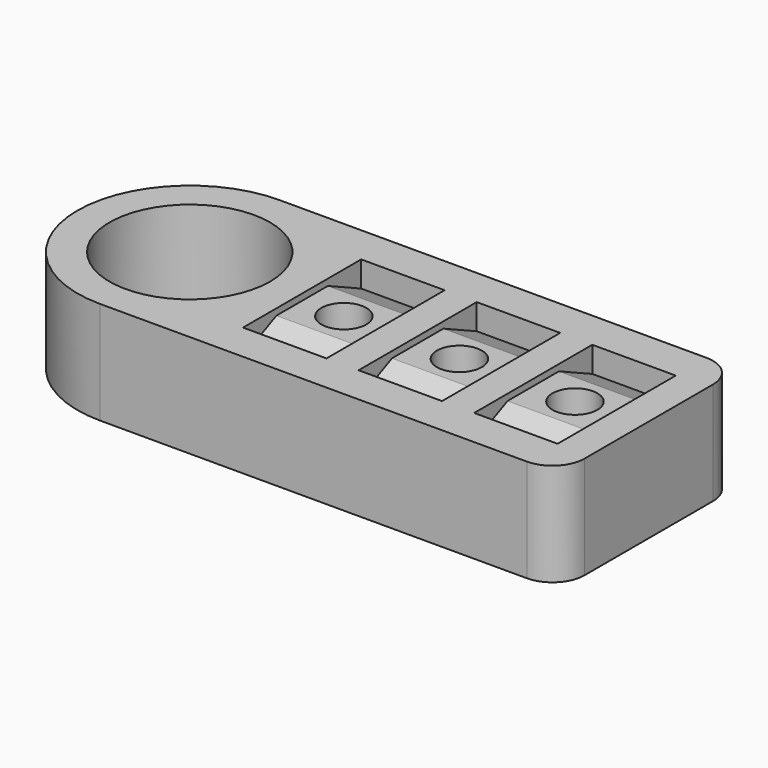
from build123d import *

# Parameters (mm, degrees)
F0_R         = 12.5
F1_DEPTH     = 16
F3_START     = -5
F3_DEPTH     = 13
F4_START     = -23
F4_DEPTH     = 13
F5_START     = -41
F5_DEPTH     = 13
F6_R         = 3.5
F7_DEPTH     = 14
F8_TEXT_SIZE = 5.5555555556
F9_DEPTH     = 1


# Not quite as in the source:
# - Text() gives the source's letters only with a copy of the font that has no kerning and outlines rounded to 1/6400 em; it was checked with that copy


with BuildPart() as f1:
    # F0 (on Top) → F1 (new body)
    with BuildSketch(Plane.XY):
        with BuildLine():
            ThreePointArc((0, 17.5), (5.1256313292, 5.1256313292), (17.5, 0))
            Line((17.5, 0), (84, 0))
            ThreePointArc((84, 0), (87.5355339059, 1.4644660941), (89, 5))
            Line((89, 5), (89, 30))
            ThreePointArc((89, 30), (87.5355339059, 33.5355339059), (84, 35))
            Line((84, 35), (17.5, 35))
            ThreePointArc((17.5, 35), (5.1256313292, 29.8743686708), (0, 17.5))
        make_face()
        with Locations((17.5, 17.5)):
            Circle(F0_R, mode=Mode.SUBTRACT)
    extrude(amount=F1_DEPTH)

    # F2 (on face) → F3 (cut)
    with BuildSketch(Plane.YZ.offset(89).offset(F3_START)):
        Polygon((6, 12), (12.5, 15), (22.5, 15), (29, 12), (29, 16), (6, 16), align=None)
    extrude(amount=-F3_DEPTH, mode=Mode.SUBTRACT)

    # F2 (on face) → F4 (cut)
    with BuildSketch(Plane.YZ.offset(89).offset(F4_START)):
        Polygon((6, 12), (12.5, 15), (22.5, 15), (29, 12), (29, 16), (6, 16), align=None)
    extrude(amount=-F4_DEPTH, mode=Mode.SUBTRACT)

    # F2 (on face) → F5 (cut)
    with BuildSketch(Plane.YZ.offset(89).offset(F5_START)):
        Polygon((6, 12), (12.5, 15), (22.5, 15), (29, 12), (29, 16), (6, 16), align=None)
    extrude(amount=-F5_DEPTH, mode=Mode.SUBTRACT)

    # F6 (on face) → F7 (cut)
    with BuildSketch(Plane.XY.offset(15)):
        with Locations((41.5, 17.5)):
            Circle(F6_R)
        with Locations((59.5, 17.5)):
            Circle(F6_R)
        with Locations((77.5, 17.5)):
            Circle(F6_R)
    extrude(amount=-F7_DEPTH, mode=Mode.SUBTRACT)

    # F8 (on face) → F9 (cut)
    with BuildSketch(Plane(origin=(0, 0, 0), x_dir=(1, 0, 0), z_dir=(0, 0, -1))):
        with Locations((30, -9)):
            Text('848', F8_TEXT_SIZE, font='Open Sans', text_align=(TextAlign.LEFT, TextAlign.BOTTOM))
    extrude(amount=-F9_DEPTH, mode=Mode.SUBTRACT)


solid = f1.part
